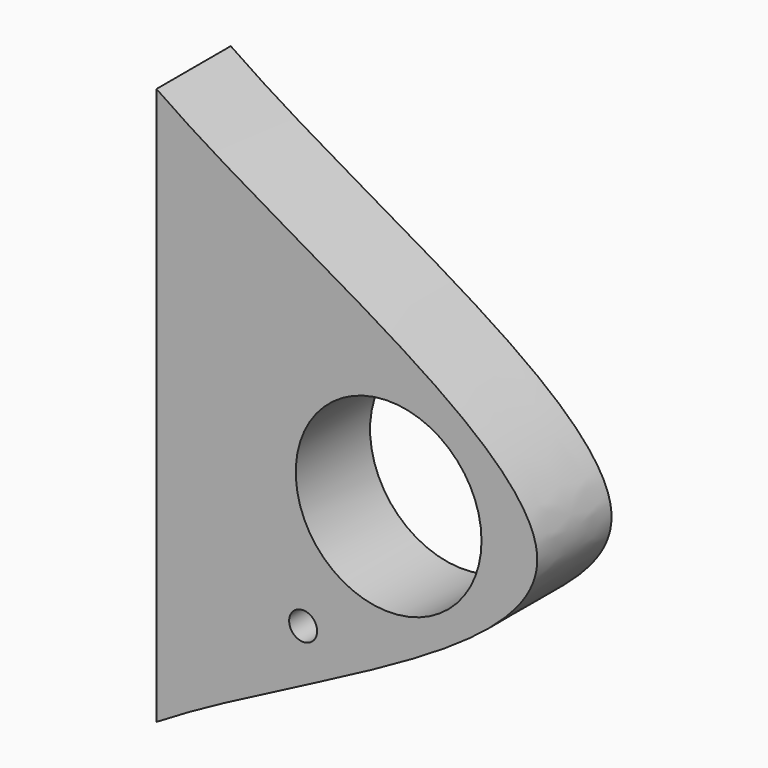
from build123d import *

# Parameters (mm, degrees)
F0_R     = 1.9127396408
F0_R_2   = 12.7
F1_DEPTH = 12.7
F2_DEPTH = 25.4


# Not quite as in the source:
# - the program builds the solid bodies; features that only make, move or delete a surface that nothing else refers to are left out


with BuildPart() as f1:
    # F0 (on Front) → F1 (new body, symmetric)
    with BuildSketch(Plane.XZ):
        with BuildLine():
            add(Edge.make_bspline(
                [(-52.07, 39.934753072), (-32.7317643122, 26.4345029642), (32.8229777519, -0.6113982397), (-32.9020863732, -24.3593875318), (-52.07, -36.265246928)],
                knots=[0, 0, 0, 0, 0.5041961308, 1, 1, 1, 1], degree=3))
            Line((-52.07, 39.934753072), (-52.07, -36.265246928))
        make_face()
        with Locations((-32.0125967264, -18.1999988854)):
            Circle(F0_R, mode=Mode.SUBTRACT)
        with Locations((-20.32, 0)):
            Circle(F0_R_2, mode=Mode.SUBTRACT)
    extrude(amount=F1_DEPTH, both=True)

    # F0 (on Front) → F2 (cut)
    with BuildSketch(Plane.XZ):
        with BuildLine():
            add(Edge.make_bspline(
                [(-52.07, 39.934753072), (-32.7317643122, 26.4345029642), (32.8229777519, -0.6113982397), (-32.9020863732, -24.3593875318), (-52.07, -36.265246928)],
                knots=[0, 0, 0, 0, 0.5041961308, 1, 1, 1, 1], degree=3))
            Line((-52.07, 39.934753072), (-52.07, -36.265246928))
        make_face()
        with Locations((-32.0125967264, -18.1999988854)):
            Circle(F0_R, mode=Mode.SUBTRACT)
        with Locations((-20.32, 0)):
            Circle(F0_R_2, mode=Mode.SUBTRACT)
    extrude(amount=-F2_DEPTH, mode=Mode.SUBTRACT)


solid = f1.part
